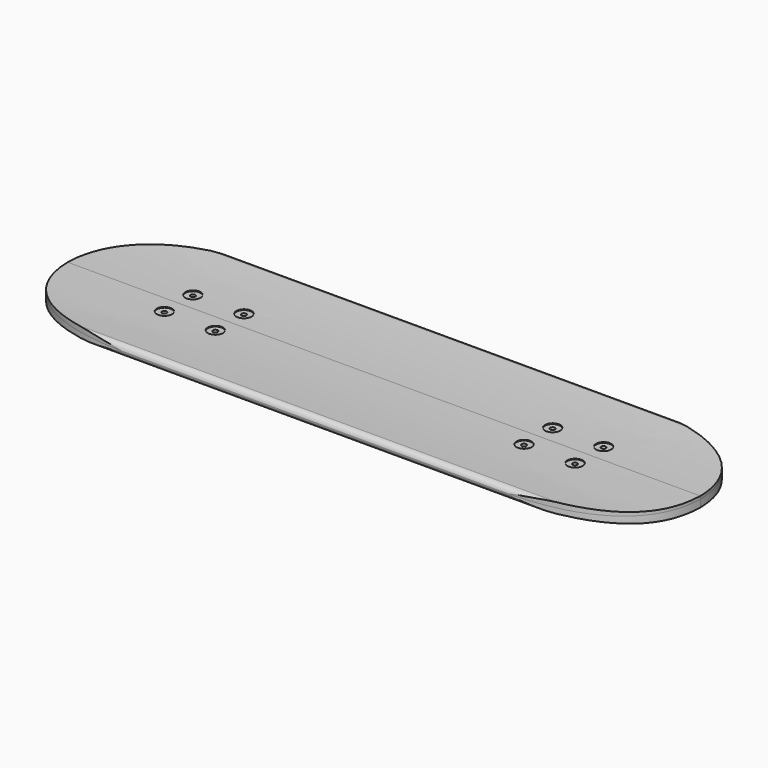
from build123d import *

# Parameters (mm, degrees)
F1_DEPTH      = 787.4
F3_DEPTH      = 50.8
F3_DEPTH_BACK = 50.8
F4_R          = 2.4892
F5_DEPTH      = 9.1599500769
F5_DEPTH_BACK = 6.3510001
F6_R          = 2.9464
F6_R_2        = 2.9718
F7_DEPTH      = 6.35
F7_DEPTH_BACK = 0.79375
F9_START      = 2.70002
F8_R          = 9.525
F9_DEPTH      = 0.9652


# Not quite as in the source:
# - a feature names something its author has since deleted; it is built from what else it names


with BuildPart() as f1:
    # F0 (on Right) → F1 (new body)
    with BuildSketch(Plane.YZ):
        with BuildLine():
            ThreePointArc((101.6, -6.35), (106.0901280605, -4.4901280605), (107.95, 0))
            ThreePointArc((107.95, 0), (106.0901280605, 4.4901280605), (101.6, 6.35))
            add(Edge.make_bspline(
                [(101.6, 6.35), (68.3791562915, 3.4076566808), (34.5582813025, 3.6700451747), (0, 3.5626797471)],
                knots=[0, 0, 0, 0, 101.6382268351, 101.6382268351, 101.6382268351, 101.6382268351], degree=3))
            add(Edge.make_bspline(
                [(-101.6, 6.35), (-68.3791562915, 3.4076566808), (-34.5582813025, 3.6700451747), (0, 3.5626797471)],
                knots=[0, 0, 0, 0, 101.6382268351, 101.6382268351, 101.6382268351, 101.6382268351], degree=3))
            ThreePointArc((-101.6, 6.35), (-106.0901280605, 4.4901280605), (-107.95, 0))
            ThreePointArc((-107.95, 0), (-106.0901280605, -4.4901280605), (-101.6, -6.35))
            add(Edge.make_bspline(
                [(-101.6, -6.35), (-75.3396605721, -8.603187674), (-49.8510954752, -9.4097596525), (-23.7861258961, -9.0927485042)],
                knots=[0, 0, 0, 0, 78.0691539893, 78.0691539893, 78.0691539893, 78.0691539893], degree=3))
            add(Edge.make_bspline(
                [(-23.7861258961, -9.0927485042), (-15.9222260953, -8.997105043), (-8.0058589787, -8.799187237), (0, -8.5078664124)],
                knots=[78.0691539893, 78.0691539893, 78.0691539893, 78.0691539893, 101.622912709, 101.622912709, 101.622912709, 101.622912709], degree=3))
            add(Edge.make_bspline(
                [(23.7861258961, -9.0927485042), (15.9222260953, -8.997105043), (8.0058589787, -8.799187237), (0, -8.5078664124)],
                knots=[78.0691539893, 78.0691539893, 78.0691539893, 78.0691539893, 101.622912709, 101.622912709, 101.622912709, 101.622912709], degree=3))
            add(Edge.make_bspline(
                [(101.6, -6.35), (75.3396605721, -8.603187674), (49.8510954752, -9.4097596525), (23.7861258961, -9.0927485042)],
                knots=[0, 0, 0, 0, 78.0691539893, 78.0691539893, 78.0691539893, 78.0691539893], degree=3))
        make_face()
        with BuildLine():
            Line((-23.7861258961, -9.0927485042), (23.7861258961, -9.0927485042))
            add(Edge.make_bspline(
                [(23.7861258961, -9.0927485042), (15.9222260953, -8.997105043), (8.0058589787, -8.799187237), (0, -8.5078664124)],
                knots=[78.0691539893, 78.0691539893, 78.0691539893, 78.0691539893, 101.622912709, 101.622912709, 101.622912709, 101.622912709], degree=3))
            add(Edge.make_bspline(
                [(-23.7861258961, -9.0927485042), (-15.9222260953, -8.997105043), (-8.0058589787, -8.799187237), (0, -8.5078664124)],
                knots=[78.0691539893, 78.0691539893, 78.0691539893, 78.0691539893, 101.622912709, 101.622912709, 101.622912709, 101.622912709], degree=3))
        make_face()
    extrude(amount=F1_DEPTH)

    # F2 (on Top) → F3 (cut, two sides)
    with BuildSketch(Plane.XY) as f3_sk:
        with BuildLine():
            add(Edge.make_bspline(
                [(0, 0), (1.2114918931, -65.1885116203), (55.3569495678, -107.9504415393), (161.1240506172, -108.0528050661)],
                knots=[0, 0, 0, 0, 194.0009494048, 194.0009494048, 194.0009494048, 194.0009494048], degree=3))
            add(Edge.make_bspline(
                [(0, 0), (1.2114918931, 65.1885116203), (55.3569495678, 107.9504415393), (161.1240506172, 108.0528050661)],
                knots=[0, 0, 0, 0, 194.0009494048, 194.0009494048, 194.0009494048, 194.0009494048], degree=3))
            Line((161.1240506172, 108.0528050661), (161.1240506172, 193.4350430965))
            Line((161.1240506172, 193.4350430965), (-168.9135879278, 193.4350430965))
            Line((-168.9135879278, 193.4350430965), (-168.9135879278, -217.4469530582))
            Line((-168.9135879278, -217.4469530582), (161.1240506172, -217.4469530582))
            Line((161.1240506172, -217.4469530582), (161.1240506172, -108.0528050661))
        make_face()
        with BuildLine():
            Line((626.2758970261, -108.0528050661), (626.2758970261, -217.4469530582))
            Line((626.2758970261, -217.4469530582), (956.3135355711, -217.4469530582))
            Line((956.3135355711, -217.4469530582), (956.3135355711, 193.4350430965))
            Line((956.3135355711, 193.4350430965), (626.2758970261, 193.4350430965))
            Line((626.2758970261, 193.4350430965), (626.2758970261, 108.0528050661))
            add(Edge.make_bspline(
                [(787.3999476433, 0), (786.1884557502, 65.1885116203), (732.0429980755, 107.9504415393), (626.2758970261, 108.0528050661)],
                knots=[0, 0, 0, 0, 194.0009494048, 194.0009494048, 194.0009494048, 194.0009494048], degree=3))
            add(Edge.make_bspline(
                [(787.3999476433, 0), (786.1884557502, -65.1885116203), (732.0429980755, -107.9504415393), (626.2758970261, -108.0528050661)],
                knots=[0, 0, 0, 0, 194.0009494048, 194.0009494048, 194.0009494048, 194.0009494048], degree=3))
        make_face()
    extrude(amount=-F3_DEPTH, mode=Mode.SUBTRACT)
    extrude(f3_sk.sketch, amount=F3_DEPTH_BACK, mode=Mode.SUBTRACT)

    # F4 (on Top) → F5 (cut, two sides)
    with BuildSketch(Plane.XY) as f5_sk:
        with Locations((138.181137654, -22.225)):
            Circle(F4_R)
        with Locations((201.681137654, -22.225)):
            Circle(F4_R)
        with Locations((138.181137654, 22.225)):
            Circle(F4_R)
        with Locations((201.681137654, 22.225)):
            Circle(F4_R)
        with Locations((585.7188099892, 22.225)):
            Circle(F4_R)
        with Locations((585.7188099892, -22.225)):
            Circle(F4_R)
        with Locations((649.2188099892, -22.225)):
            Circle(F4_R)
        with Locations((649.2188099892, 22.225)):
            Circle(F4_R)
    extrude(amount=-F5_DEPTH, mode=Mode.SUBTRACT)
    extrude(f5_sk.sketch, amount=F5_DEPTH_BACK, mode=Mode.SUBTRACT)

    # F6 (on Top) → F7 (cut, two sides)
    with BuildSketch(Plane.XY) as f7_sk:
        with Locations((138.1544321775, 22.225)):
            Circle(F6_R)
        with Locations((201.6517895361, 22.225)):
            Circle(F6_R_2)
        with Locations((585.6845495361, 22.225)):
            Circle(F6_R_2)
        with Locations((649.1819068947, 22.225)):
            Circle(F6_R)
        with Locations((138.1544321775, -22.225)):
            Circle(F6_R)
        with Locations((201.6517895361, -22.225)):
            Circle(F6_R_2)
        with Locations((649.1819068947, -22.225)):
            Circle(F6_R)
        with Locations((585.6845495361, -22.225)):
            Circle(F6_R_2)
    extrude(amount=F7_DEPTH, mode=Mode.SUBTRACT)
    extrude(f7_sk.sketch, amount=-F7_DEPTH_BACK, mode=Mode.SUBTRACT)

    # F8 (on Top) → F9 (cut)
    with BuildSketch(Plane.XY.offset(F9_START)):
        with Locations((138.176003624, 22.225)):
            Circle(F8_R)
        with Locations((201.683623624, 22.225)):
            Circle(F8_R)
        with Locations((201.683623624, -22.225)):
            Circle(F8_R)
        with Locations((138.176003624, -22.225)):
            Circle(F8_R)
        with Locations((585.716383624, -22.225)):
            Circle(F8_R)
        with Locations((585.716383624, 22.225)):
            Circle(F8_R)
        with Locations((649.224003624, 22.225)):
            Circle(F8_R)
        with Locations((649.224003624, -22.225)):
            Circle(F8_R)
    extrude(amount=F9_DEPTH, mode=Mode.SUBTRACT)


solid = f1.part
